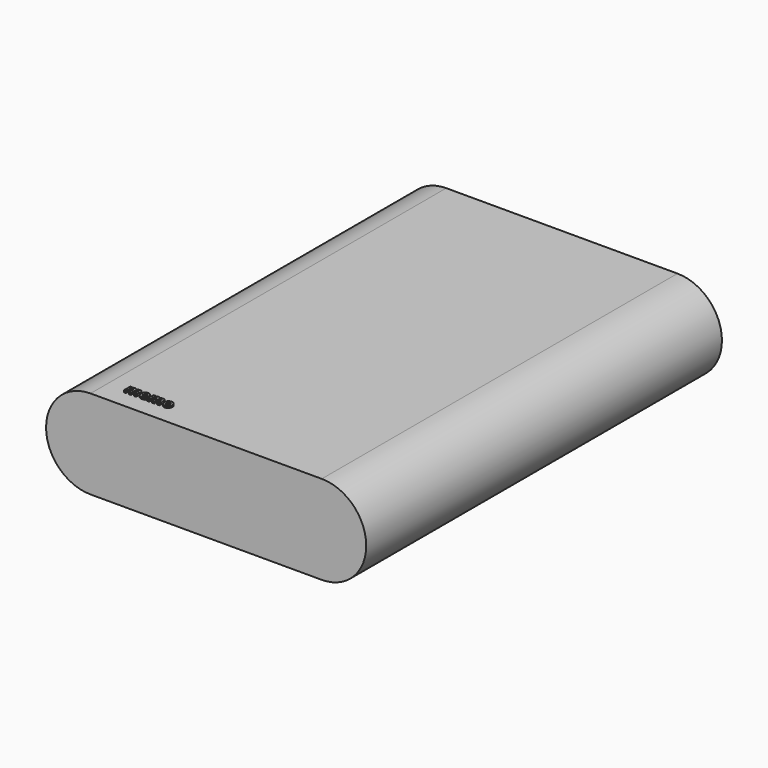
from build123d import *

# Parameters (mm, degrees)
F1_DEPTH     = 125
F2_DEPTH     = 2
F3_TEXT_SIZE = 4.1641849611
F4_DEPTH     = 0.5


# Not quite as in the source:
# - Text() gives the source's letters only with a copy of the font that has no kerning and outlines rounded to 1/6400 em; it was checked with that copy


with BuildPart() as f1:
    # F0 (on Front) → F1 (new body)
    with BuildSketch(Plane.XZ):
        with BuildLine():
            Line((32.5, 0), (-32.5, 0))
            ThreePointArc((-32.5, 0), (-45, -12.5), (-32.5, -25))
            Line((-32.5, -25), (32.5, -25))
            ThreePointArc((32.5, -25), (45, -12.5), (32.5, 0))
        make_face()
        with BuildLine():
            ThreePointArc((-32.5, -23), (-43, -12.5), (-32.5, -2))
            Line((-32.5, -2), (32.5, -2))
            ThreePointArc((32.5, -2), (43, -12.5), (32.5, -23))
            Line((32.5, -23), (-32.5, -23))
        make_face(mode=Mode.SUBTRACT)
    extrude(amount=-F1_DEPTH)

    # F0 (on Front) → F2 (join)
    with BuildSketch(Plane.XZ):
        with BuildLine():
            Line((32.5, -2), (-32.5, -2))
            ThreePointArc((-32.5, -2), (-43, -12.5), (-32.5, -23))
            Line((-32.5, -23), (32.5, -23))
            ThreePointArc((32.5, -23), (43, -12.5), (32.5, -2))
        make_face()
    extrude(amount=-F2_DEPTH)

    # F3 (on Top) → F4 (join)
    with BuildSketch(Plane.XY):
        with Locations((-27.4737280607, 5)):
            Text('memo', F3_TEXT_SIZE, font='Open Sans', font_style=FontStyle.BOLD, text_align=(TextAlign.LEFT, TextAlign.BOTTOM))
    extrude(amount=F4_DEPTH)


solid = f1.part
